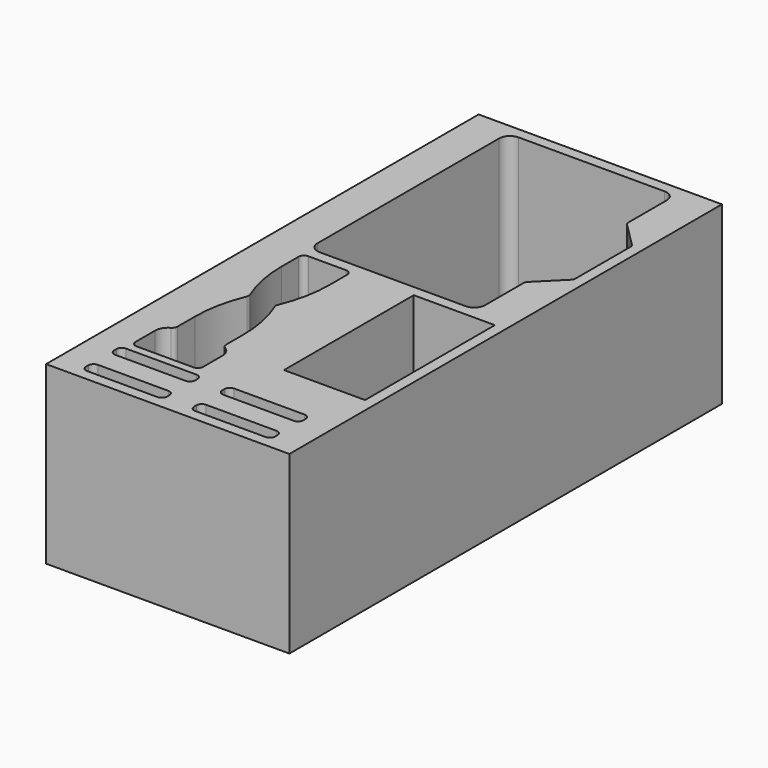
from build123d import *

# Parameters (mm, degrees)
F0_W        = 90
F0_H        = 200
F1_DEPTH    = 65
F2_W        = 62
F2_H        = 92
F2_W_2      = 30
F2_H_2      = 60
F2_H_3      = 5
F3_DEPTH    = 62
F4_R        = 4
F6_W        = 10
F6_H        = 25
F7_DEPTH    = 62
F8_T4_DEPTH = 90.2885128676
F8_T9_DEPTH = 90.2885128676
F9_R        = 2
F10_R       = 5


# Not quite as in the source:
# - a fillet or chamfer that OpenCascade refuses, or shapes differently, is made with other operations: its cross-section is extruded or revolved along the edge and cut away or added


with BuildPart() as f1:
    # F0 (on Top) → F1 (new body)
    with BuildSketch(Plane.XY):
        Rectangle(F0_W, F0_H)
    extrude(amount=F1_DEPTH)

    # F2 (on face) → F3 (cut)
    with BuildSketch(Plane.XY.offset(65)):
        with Locations((0, 50)):
            Rectangle(F2_W, F2_H)
        with Locations((26, -30)):
            Rectangle(F2_W_2, F2_H_2)
        with Locations((20, -80.5)):
            Rectangle(F2_W_2, F2_H_3)
        with Locations((20, -93.5)):
            Rectangle(F2_W_2, F2_H_3)
        with Locations((-20, -93.5)):
            Rectangle(F2_W_2, F2_H_3)
        with Locations((-20, -80.5)):
            Rectangle(F2_W_2, F2_H_3)
        with BuildLine():
            Line((-12, 0), (-30, 0))
            Line((-30, 0), (-30, -10))
            ThreePointArc((-30, -10), (-28.9453156465, -20.2154821845), (-25.8257569496, -30))
            ThreePointArc((-25.8257569496, -30), (-28.9453156465, -39.7845178155), (-30, -50))
            Line((-30, -50), (-30, -60))
            Line((-30, -60), (-12, -60))
            Line((-12, -60), (-12, -50))
            ThreePointArc((-12, -50), (-13.0546843535, -39.7845178155), (-16.1742430504, -30))
            ThreePointArc((-16.1742430504, -30), (-13.0546843535, -20.2154821845), (-12, -10))
            Line((-12, -10), (-12, 0))
        make_face()
    extrude(amount=-F3_DEPTH, mode=Mode.SUBTRACT)

    # F4
    f4_edges = [f1.edges().sort_by_distance(p)[0] for p in [
        (-31, 96, 34),
        (31, 96, 34),
        (-31, 4, 34),
        (31, 4, 34),
    ]]
    fillet(f4_edges, radius=F4_R)

    # F6 (on face) → F7 (cut, through all)
    with BuildSketch(Plane.XY.offset(65)):
        with Locations((36, 50)):
            Rectangle(F6_W, F6_H)
        Polygon((-30, -60), (-33.5, -60), (-33.5, -75), (-8.5, -75), (-8.5, -60), (-12, -60), align=None)
    extrude(amount=-F7_DEPTH, mode=Mode.SUBTRACT)

    # F8: chamfer of 11 on 2 edges, made by hand


with BuildPart() as f8_tool2:
    # F8_s3 → F8_t4 (new body)
    with BuildSketch(Plane.XY.offset(93.2885128676)):
        Polygon((42, 62.5), (31, 73.5), (31, 62.5), align=None)
    extrude(amount=-F8_T4_DEPTH)

    split(bisect_by=Plane.YZ.offset(41), keep=Keep.BOTTOM)


with BuildPart() as f1_1:
    add(f1.part)

    # F8_t1: cut F8_tool2
    add(f8_tool2.part, mode=Mode.SUBTRACT)


with BuildPart() as f8_tool7:
    # F8_s8 → F8_t9 (new body)
    with BuildSketch(Plane.XY.offset(93.2885128676)):
        Polygon((31, 26.5), (42, 37.5), (31, 37.5), align=None)
    extrude(amount=-F8_T9_DEPTH)

    split(bisect_by=Plane.YZ.offset(41), keep=Keep.BOTTOM)


with BuildPart() as f1_2:
    add(f1_1.part)

    # F8_t6: cut F8_tool7
    add(f8_tool7.part, mode=Mode.SUBTRACT)

    # F9
    f9_edges = [f1_2.edges().sort_by_distance(p)[0] for p in [
        (31, 73.5, 34),
        (41, 63.5, 34),
        (41, 36.5, 34),
        (31, 26.5, 34),
        (-30, 0, 34),
        (-12, 0, 34),
        (-16.174243, -30, 34),
        (-25.825757, -30, 34),
        (-30, -60, 34),
        (-12, -60, 34),
        (-8.5, -75, 34),
        (-33.5, -75, 34),
        (-35, -78, 34),
        (-35, -91, 34),
        (5, -91, 34),
        (5, -78, 34),
        (-5, -91, 34),
        (-5, -78, 34),
        (35, -78, 34),
        (35, -91, 34),
        (-5, -83, 34),
        (-5, -96, 34),
        (35, -96, 34),
        (35, -83, 34),
        (5, -96, 34),
        (5, -83, 34),
        (-35, -83, 34),
        (-35, -96, 34),
    ]]
    fillet(f9_edges, radius=F9_R)

    # F10
    f10_edges = [f1_2.edges().sort_by_distance(p)[0] for p in [
        (-33.5, -60, 34),
        (-8.5, -60, 34),
    ]]
    fillet(f10_edges, radius=F10_R)


solid = f1_2.part
